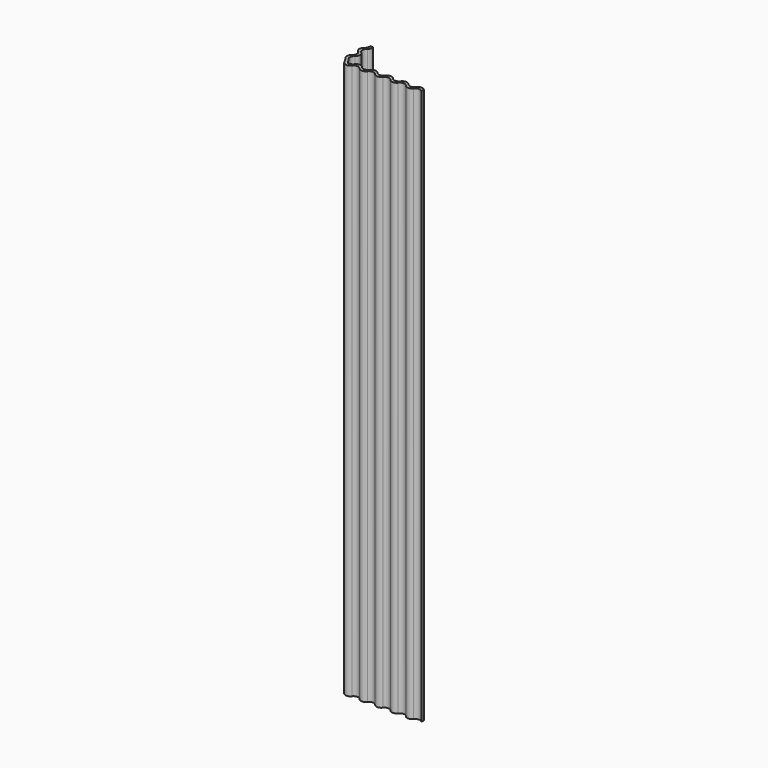
from build123d import *

# Parameters (mm, degrees)
F1_DEPTH = 144


# Not quite as in the source:
# - ends of sketch curves that miss each other by under 0.0002 mm in the source are joined


with BuildPart() as f1:
    # F0 (on Top) → F1 (new body)
    with BuildSketch(Plane.XY):
        with BuildLine():
            ThreePointArc((-9.410914, -8.92081), (-9.910914, -7.92081), (-9.410914, -6.92081))
            ThreePointArc((-9.410914, -6.92081), (-8.9764458997, -6.320228727), (-8.9585015185, -5.57919))
            Line((-8.9585015185, -5.57919), (-9.7585015185, -5.57919))
            ThreePointArc((-9.7585015185, -5.57919), (-9.7764458997, -6.320228727), (-10.210914, -6.92081))
            ThreePointArc((-10.210914, -6.92081), (-10.710914, -7.92081), (-10.210914, -8.92081))
            ThreePointArc((-10.210914, -8.92081), (-9.710914, -9.92081), (-10.210914, -10.92081))
            ThreePointArc((-10.210914, -10.92081), (-10.7014813869, -11.7675371761), (-10.4317470851, -12.708200069))
            ThreePointArc((-10.4317470851, -12.708200069), (-10.3460553781, -12.8219008439), (-10.2686699127, -12.9414099478))
            Line((-10.2686699127, -12.9414099478), (-9.289086, -14.57919))
            ThreePointArc((-9.289086, -14.57919), (-8.289086, -15.07919), (-7.289086, -14.57919))
            ThreePointArc((-7.289086, -14.57919), (-6.289086, -14.07919), (-5.289086, -14.57919))
            ThreePointArc((-5.289086, -14.57919), (-4.289086, -15.07919), (-3.289086, -14.57919))
            ThreePointArc((-3.289086, -14.57919), (-2.289086, -14.07919), (-1.289086, -14.57919))
            ThreePointArc((-1.289086, -14.57919), (-0.289086, -15.07919), (0.710914, -14.57919))
            ThreePointArc((0.710914, -14.57919), (1.710914, -14.07919), (2.710914, -14.57919))
            ThreePointArc((2.710914, -14.57919), (3.710914, -15.07919), (4.710914, -14.57919))
            ThreePointArc((4.710914, -14.57919), (5.710914, -14.07919), (6.710914, -14.57919))
            ThreePointArc((6.710914, -14.57919), (7.710914, -15.07919), (8.710914, -14.57919))
            ThreePointArc((8.710914, -14.57919), (9.710914, -14.07919), (10.710914, -14.57919))
            Line((10.710914, -14.57919), (10.710914, -13.77919))
            ThreePointArc((10.710914, -13.77919), (9.710914, -13.27919), (8.710914, -13.77919))
            ThreePointArc((8.710914, -13.77919), (7.710914, -14.27919), (6.710914, -13.77919))
            ThreePointArc((6.710914, -13.77919), (5.710914, -13.27919), (4.710914, -13.77919))
            ThreePointArc((4.710914, -13.77919), (3.710914, -14.27919), (2.710914, -13.77919))
            ThreePointArc((2.710914, -13.77919), (1.710914, -13.27919), (0.710914, -13.77919))
            ThreePointArc((0.710914, -13.77919), (-0.289086, -14.27919), (-1.289086, -13.77919))
            ThreePointArc((-1.289086, -13.77919), (-2.289086, -13.27919), (-3.289086, -13.77919))
            ThreePointArc((-3.289086, -13.77919), (-4.289086, -14.27919), (-5.289086, -13.77919))
            ThreePointArc((-5.289086, -13.77919), (-6.289086, -13.27919), (-7.289086, -13.77919))
            ThreePointArc((-7.289086, -13.77919), (-7.7801177198, -14.1708779126), (-8.3996640349, -14.2742893929))
            ThreePointArc((-8.3996640349, -14.2742893929), (-8.6183007719, -14.2015740347), (-8.7811153103, -14.0385371912))
            Line((-8.7811153103, -14.0385371912), (-9.438132, -12.972224))
            ThreePointArc((-9.438132, -12.972224), (-9.5218512465, -12.8471466938), (-9.6147395194, -12.7287194399))
            ThreePointArc((-9.6147395194, -12.7287194399), (-9.9030448701, -11.7807710715), (-9.410914, -10.92081))
            ThreePointArc((-9.410914, -10.92081), (-8.910914, -9.92081), (-9.410914, -8.92081))
        make_face()
    extrude(amount=F1_DEPTH)


solid = f1.part
